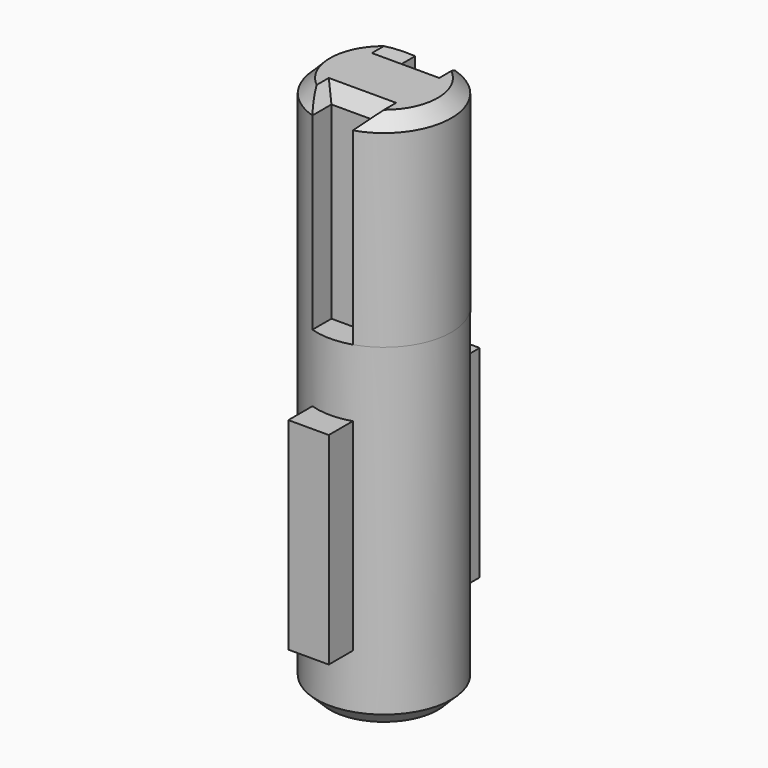
from build123d import *

# Parameters (mm, degrees)
F0_R         = 5
F1_DEPTH     = 5
F3_DEPTH     = 15
F5_DEPTH     = 5
F7_DEPTH     = 15
F8_T1_DEPTH  = 4.3413789951
F8_T3_DEPTH  = 3
F8_T5_DEPTH  = 4.3413789951
F8_T10_ANGLE = 204.0849815342
F8_T12_ANGLE = 204.0849815342
F8_T17_DEPTH = 6.913061983
F8_T21_DEPTH = 5.571682988
F8_T28_DEPTH = 6.913061983
F8_T32_DEPTH = 5.571682988
F8_T39_DEPTH = 6.913061983
F8_T43_DEPTH = 5.571682988
F8_T50_DEPTH = 5.571682988
F8_T54_DEPTH = 6.913061983


# Not quite as in the source:
# - a fillet or chamfer that OpenCascade refuses, or shapes differently, is made with other operations: its cross-section is extruded or revolved along the edge and cut away or added


with BuildPart() as f1:
    # F0 (on Top) → F1 (new body)
    with BuildSketch(Plane.XY):
        Circle(F0_R)
    extrude(amount=F1_DEPTH)

    # F2 (on face) → F3 (join)
    with BuildSketch(Plane.XY.offset(5)):
        with BuildLine():
            Line((-1.5, 7), (-1.5, 4.7696960071))
            ThreePointArc((-1.5, 4.7696960071), (-5, 0), (-1.5, -4.7696960071))
            Line((-1.5, -4.7696960071), (-1.5, -7))
            Line((-1.5, -7), (1.5, -7))
            Line((1.5, -7), (1.5, -4.7696960071))
            ThreePointArc((1.5, -4.7696960071), (5, 0), (1.5, 4.7696960071))
            Line((1.5, 4.7696960071), (1.5, 7))
            Line((1.5, 7), (-1.5, 7))
        make_face()
    extrude(amount=F3_DEPTH)

    # F4 (on face) → F5 (join)
    with BuildSketch(Plane.XY.offset(20)):
        with BuildLine():
            ThreePointArc((1.5, -4.7696960071), (4.0311288741, -2.9580398915), (5, 0))
            ThreePointArc((5, 0), (4.0311288741, 2.9580398915), (1.5, 4.7696960071))
            ThreePointArc((1.5, 4.7696960071), (0, 5), (-1.5, 4.7696960071))
            ThreePointArc((-1.5, 4.7696960071), (-5, 0), (-1.5, -4.7696960071))
            ThreePointArc((-1.5, -4.7696960071), (0, -5), (1.5, -4.7696960071))
        make_face()
    extrude(amount=F5_DEPTH)

    # F6 (on face) → F7 (join)
    with BuildSketch(Plane.XY.offset(25)):
        with BuildLine():
            Line((1.5, -3), (1.5, -4.7696960071))
            ThreePointArc((1.5, -4.7696960071), (5, 0), (1.5, 4.7696960071))
            Line((1.5, 4.7696960071), (1.5, 3))
            Line((1.5, 3), (-1.5, 3))
            Line((-1.5, 3), (-1.5, 4.7696960071))
            ThreePointArc((-1.5, 4.7696960071), (-5, 0), (-1.5, -4.7696960071))
            Line((-1.5, -4.7696960071), (-1.5, -3))
            Line((-1.5, -3), (1.5, -3))
        make_face()
    extrude(amount=F7_DEPTH)

    # F8: chamfer of 1 on 9 edges, made by hand

    # F8_s2 → F8_t1 (cut)
    with BuildSketch(Plane.XZ.offset(3)):
        Polygon((-2.5, 40), (-1.5, 39), (-1.5, 40), align=None)
        Polygon((1.5, 39), (2.5, 40), (1.5, 40), align=None)
    extrude(amount=F8_T1_DEPTH, mode=Mode.SUBTRACT)

    # F8_s4 → F8_t3 (cut)
    with BuildSketch(Plane.YZ.offset(-1.5)):
        Polygon((-2, 40), (-3, 39), (-3, 40), align=None)
        Polygon((2, 40), (3, 39), (3, 40), align=None)
    extrude(amount=F8_T3_DEPTH, mode=Mode.SUBTRACT)

    # F8_s6 → F8_t5 (cut)
    with BuildSketch(Plane.XZ.offset(-7.3413789951)):
        Polygon((1.5, 39), (2.5, 40), (1.5, 40), align=None)
        Polygon((-2.5, 40), (-1.5, 39), (-1.5, 40), align=None)
    extrude(amount=F8_T5_DEPTH, mode=Mode.SUBTRACT)

    # F8_s7 → F8_t8 (revolve, cut)
    with BuildSketch(Plane.XZ):
        Polygon((5, 1), (4, 0), (5, 0), align=None)
    revolve(axis=Axis((0, 0, 0), (0, 0, 1)), mode=Mode.SUBTRACT)

    # F8_s9 → F8_t10 (revolve, cut)
    with BuildSketch(Plane(origin=(0, 0, 0), x_dir=(0, 0, 1), z_dir=(-0.9779931437, 0.2086370315, 0))):
        Polygon((39, -5), (40, -4), (40, -5), align=None)
    revolve(axis=Axis((0, 0, 40), (0, 0, 1)), revolution_arc=F8_T10_ANGLE, mode=Mode.SUBTRACT)

    # F8_s11 → F8_t12 (revolve, cut)
    with BuildSketch(Plane(origin=(0, 0, 0), x_dir=(0, 0, 1), z_dir=(0.9779931437, -0.2086370315, 0))):
        Polygon((39, -5), (40, -4), (40, -5), align=None)
    revolve(axis=Axis((0, 0, 40), (0, 0, 1)), revolution_arc=F8_T12_ANGLE, mode=Mode.SUBTRACT)


with BuildPart() as f8_tool15:
    # F8_s16 → F8_t17 (new body)
    with BuildSketch(Plane.XZ.offset(7.3413789951)):
        Polygon((-2.5, 40), (-1.5, 39), (-1.5, 40), align=None)
    extrude(amount=-F8_T17_DEPTH)

    split(bisect_by=Plane.XZ.offset(3), keep=Keep.BOTTOM)


with BuildPart() as f8_tool19:
    # F8_s20 → F8_t21 (new body)
    with BuildSketch(Plane.YZ.offset(-4.071682988)):
        Polygon((-2, 40), (-3, 39), (-3, 40), align=None)
    extrude(amount=F8_T21_DEPTH)

    split(bisect_by=Plane.YZ.offset(-1.5), keep=Keep.BOTTOM)


with BuildPart() as f8_tool15_1:
    add(f8_tool15.part)

    # F8_t23: intersect F8_tool19
    add(f8_tool19.part, mode=Mode.INTERSECT)


with BuildPart() as f1_1:
    add(f1.part)

    # F8_t13: cut F8_tool15
    add(f8_tool15_1.part, mode=Mode.SUBTRACT)


with BuildPart() as f8_tool26:
    # F8_s27 → F8_t28 (new body)
    with BuildSketch(Plane.XZ.offset(0.428317012)):
        Polygon((1.5, 39), (2.5, 40), (1.5, 40), align=None)
    extrude(amount=F8_T28_DEPTH)

    split(bisect_by=Plane.XZ.offset(3), keep=Keep.BOTTOM)


with BuildPart() as f8_tool30:
    # F8_s31 → F8_t32 (new body)
    with BuildSketch(Plane.YZ.offset(-1.5)):
        Polygon((-2, 40), (-3, 39), (-3, 40), align=None)
    extrude(amount=F8_T32_DEPTH)

    split(bisect_by=Plane.YZ.offset(1.5), keep=Keep.TOP)


with BuildPart() as f8_tool26_1:
    add(f8_tool26.part)

    # F8_t34: intersect F8_tool30
    add(f8_tool30.part, mode=Mode.INTERSECT)


with BuildPart() as f1_2:
    add(f1_1.part)

    # F8_t24: cut F8_tool26
    add(f8_tool26_1.part, mode=Mode.SUBTRACT)


with BuildPart() as f8_tool37:
    # F8_s38 → F8_t39 (new body)
    with BuildSketch(Plane.XZ.offset(-7.3413789951)):
        Polygon((1.5, 39), (2.5, 40), (1.5, 40), align=None)
    extrude(amount=F8_T39_DEPTH)

    split(bisect_by=Plane.XZ.offset(-3), keep=Keep.TOP)


with BuildPart() as f8_tool41:
    # F8_s42 → F8_t43 (new body)
    with BuildSketch(Plane.YZ.offset(4.071682988)):
        Polygon((2, 40), (3, 39), (3, 40), align=None)
    extrude(amount=-F8_T43_DEPTH)

    split(bisect_by=Plane.YZ.offset(1.5), keep=Keep.TOP)


with BuildPart() as f8_tool37_1:
    add(f8_tool37.part)

    # F8_t45: intersect F8_tool41
    add(f8_tool41.part, mode=Mode.INTERSECT)


with BuildPart() as f1_3:
    add(f1_2.part)

    # F8_t35: cut F8_tool37
    add(f8_tool37_1.part, mode=Mode.SUBTRACT)


with BuildPart() as f8_tool48:
    # F8_s49 → F8_t50 (new body)
    with BuildSketch(Plane.YZ.offset(1.5)):
        Polygon((2, 40), (3, 39), (3, 40), align=None)
    extrude(amount=-F8_T50_DEPTH)

    split(bisect_by=Plane.YZ.offset(-1.5), keep=Keep.BOTTOM)


with BuildPart() as f8_tool52:
    # F8_s53 → F8_t54 (new body)
    with BuildSketch(Plane.XZ.offset(-0.428317012)):
        Polygon((-2.5, 40), (-1.5, 39), (-1.5, 40), align=None)
    extrude(amount=-F8_T54_DEPTH)

    split(bisect_by=Plane.XZ.offset(-3), keep=Keep.TOP)


with BuildPart() as f8_tool48_1:
    add(f8_tool48.part)

    # F8_t56: intersect F8_tool52
    add(f8_tool52.part, mode=Mode.INTERSECT)


with BuildPart() as f1_4:
    add(f1_3.part)

    # F8_t46: cut F8_tool48
    add(f8_tool48_1.part, mode=Mode.SUBTRACT)


solid = f1_4.part
